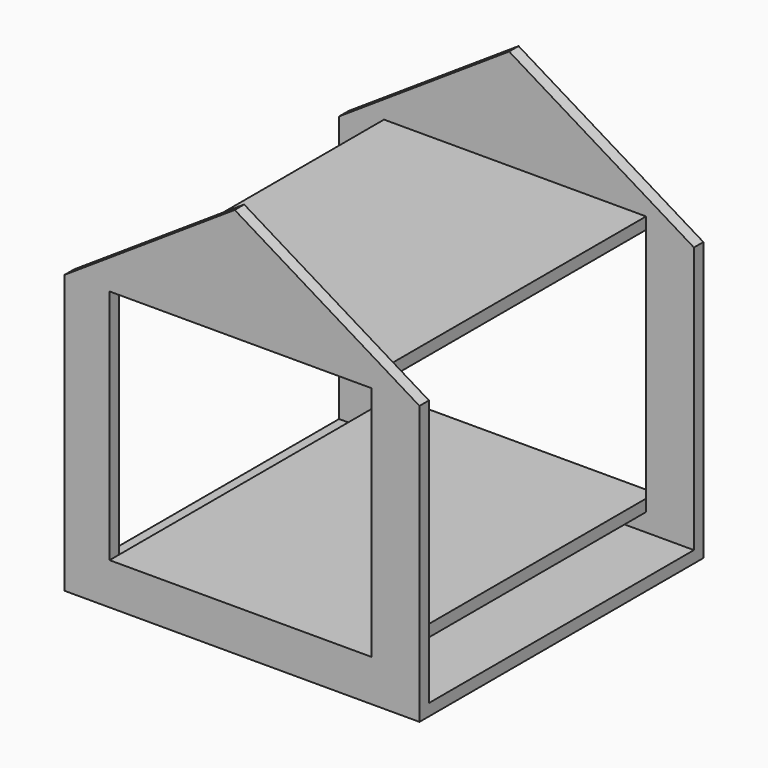
from build123d import *

# Parameters (mm, degrees)
F0_W     = 10.2729936957
F0_H     = 50.8
F0_W_2   = 9.6539677948
F1_DEPTH = 76.2
F2_T     = 2.54


# Not quite as in the source:
# - a shell that OpenCascade refuses in one call is made with other operations: the cavity is built on its own and cut out


with BuildPart() as f1:
    # F0 (on Front) → F1 (new body)
    with BuildSketch(Plane.XZ):
        Polygon((-4.9094697461, 50.2964220941), (-41.4324142039, 26.1541400105), (-31.7784464091, 26.1541400105), (24.4945921004, 26.1541400105), (34.7675857961, 26.1541400105), align=None)
        with Locations((29.6310889482, 0.7541400105)):
            Rectangle(F0_W, F0_H)
        with Locations((-36.6054303065, 0.7541400105)):
            Rectangle(F0_W_2, F0_H)
        Polygon((-31.7784464091, -24.6458599895), (-41.4324142039, -24.6458599895), (-41.4324142039, -33.582534641), (34.7675857961, -33.582534641), (34.7675857961, -24.6458599895), (24.4945921004, -24.6458599895), align=None)
    extrude(amount=F1_DEPTH)

    # F2: shell of thickness 2.54, made by hand


with BuildPart() as f2_core1:
    # F2_t2: copy of F1
    add(f1.part)

    # the walls: a layer under each face that stays
    f2_faces = [f2_core1.faces().sort_by_distance(p)[0] for p in [
        (-3.3324142039, -38.1, -33.582534641),
        (-3.6419271544, -38.1, 26.1541400105),
        (-3.6419271544, -38.1, -24.6458599895),
        (-3.3324142039, 0, 36.3165959716),
        (-3.3324142039, -76.2, 36.3165959716),
    ]]
    thicken(f2_faces, amount=-F2_T, mode=Mode.SUBTRACT)


with BuildPart() as f1_1:
    add(f1.part)

    # what is left inside the walls is the cavity
    f2_cavity = [f2_core1.part.solids().sort_by_distance(p)[0] for p in [
        (-3.332414, -49.953333, -31.017135),
    ]]
    add(f2_cavity, mode=Mode.SUBTRACT)


solid = f1_1.part
